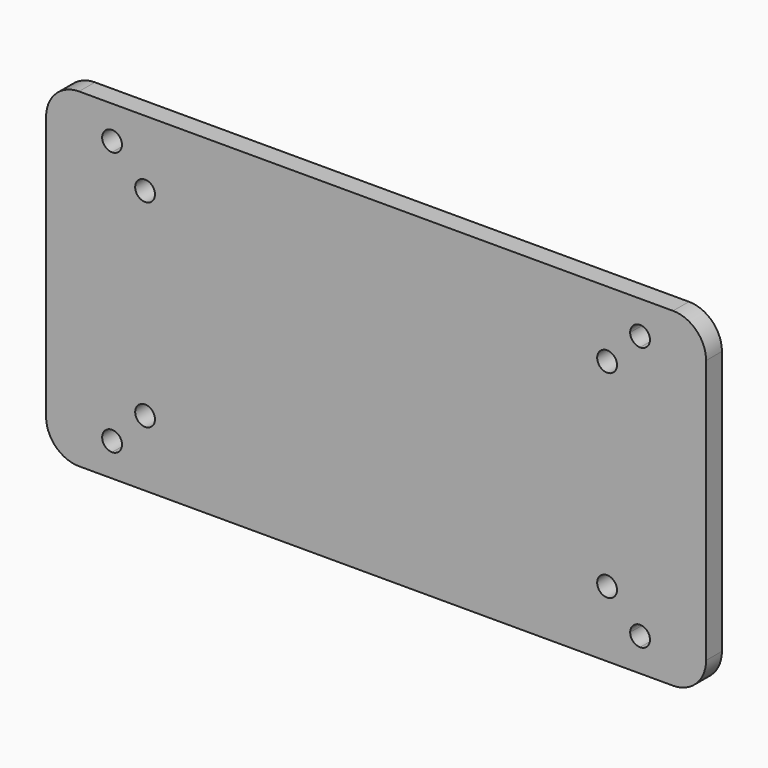
from build123d import *

# Parameters (mm, degrees)
F1_R     = 1.5
F1_R_2   = 12.8016
F2_DEPTH = 3
F3_DEPTH = 3


# Not quite as in the source:
# - a feature names something its author has since deleted; it is built from what else it names


with BuildPart() as f2:
    # F1 (on Front) → F2 (new body)
    with BuildSketch(Plane.XZ):
        with BuildLine():
            ThreePointArc((-79.8984, -48.3984), (-78.8377398282, -48.8377398282), (-78.3984, -49.8984))
            Line((-78.3984, -49.8984), (-1.3984, -49.8984))
            ThreePointArc((-1.3984, -49.8984), (-0.9590601718, -48.8377398282), (0.1016, -48.3984))
            Line((0.1016, -48.3984), (0.1016, -11.3984))
            ThreePointArc((0.1016, -11.3984), (-0.9590601718, -10.9590601718), (-1.3984, -9.8984))
            Line((-1.3984, -9.8984), (-78.3984, -9.8984))
            ThreePointArc((-78.3984, -9.8984), (-78.8377398282, -10.9590601718), (-79.8984, -11.3984))
            Line((-79.8984, -11.3984), (-79.8984, -48.3984))
        make_face()
        with Locations((-74.8984, -44.8984)):
            Circle(F1_R, mode=Mode.SUBTRACT)
        with BuildLine():
            ThreePointArc((-35.3196263313, -48.5484), (-35.6125195501, -49.2555067812), (-36.3196263313, -49.5484))
            Line((-36.3196263313, -49.5484), (-47.2771736687, -49.5484))
            ThreePointArc((-47.2771736687, -49.5484), (-47.9842804499, -49.2555067812), (-48.2771736687, -48.5484))
            Line((-48.2771736687, -48.5484), (-48.2771736687, -36.5484))
            ThreePointArc((-48.2771736687, -36.5484), (-47.9842804499, -35.8412932188), (-47.2771736687, -35.5484))
            Line((-47.2771736687, -35.5484), (-36.3196263313, -35.5484))
            ThreePointArc((-36.3196263313, -35.5484), (-35.6125195501, -35.8412932188), (-35.3196263313, -36.5484))
            Line((-35.3196263313, -36.5484), (-35.3196263313, -48.5484))
        make_face(mode=Mode.SUBTRACT)
        with Locations((-64.6584, -30.8484)):
            Circle(F1_R_2, mode=Mode.SUBTRACT)
        with Locations((-4.8984, -44.8984)):
            Circle(F1_R, mode=Mode.SUBTRACT)
        with Locations((-74.8984, -14.8984)):
            Circle(F1_R, mode=Mode.SUBTRACT)
        with BuildLine():
            ThreePointArc((-35.3196263313, -23.1484), (-35.6125195501, -23.8555067812), (-36.3196263313, -24.1484))
            Line((-36.3196263313, -24.1484), (-47.2771736687, -24.1484))
            ThreePointArc((-47.2771736687, -24.1484), (-47.9842804499, -23.8555067812), (-48.2771736687, -23.1484))
            Line((-48.2771736687, -23.1484), (-48.2771736687, -11.1484))
            ThreePointArc((-48.2771736687, -11.1484), (-47.9842804499, -10.4412932188), (-47.2771736687, -10.1484))
            Line((-47.2771736687, -10.1484), (-36.3196263313, -10.1484))
            ThreePointArc((-36.3196263313, -10.1484), (-35.6125195501, -10.4412932188), (-35.3196263313, -11.1484))
            Line((-35.3196263313, -11.1484), (-35.3196263313, -23.1484))
        make_face(mode=Mode.SUBTRACT)
        with BuildLine():
            ThreePointArc((-24.0503456444, -32.5784), (-24.3432388632, -33.2855067812), (-25.0503456444, -33.5784))
            Line((-25.0503456444, -33.5784), (-30.0664543556, -33.5784))
            ThreePointArc((-30.0664543556, -33.5784), (-30.7735611368, -33.2855067812), (-31.0664543556, -32.5784))
            Line((-31.0664543556, -32.5784), (-31.0664543556, -26.5784))
            ThreePointArc((-31.0664543556, -26.5784), (-30.7735611368, -25.8712932188), (-30.0664543556, -25.5784))
            Line((-30.0664543556, -25.5784), (-25.0503456444, -25.5784))
            ThreePointArc((-25.0503456444, -25.5784), (-24.3432388632, -25.8712932188), (-24.0503456444, -26.5784))
            Line((-24.0503456444, -26.5784), (-24.0503456444, -32.5784))
        make_face(mode=Mode.SUBTRACT)
        with BuildLine():
            ThreePointArc((-20.0169235468, -20.9634935707), (-19.724030328, -20.2563867895), (-19.0169235468, -19.9634935707))
            Line((-19.0169235468, -19.9634935707), (-13.3099917546, -19.9634935707))
            ThreePointArc((-13.3099917546, -19.9634935707), (-12.6028849734, -20.2563867895), (-12.3099917546, -20.9634935707))
            Line((-12.3099917546, -20.9634935707), (-12.3099917546, -38.3518991768))
            ThreePointArc((-12.3099917546, -38.3518991768), (-12.6028849734, -39.059005958), (-13.3099917546, -39.3518991768))
            Line((-13.3099917546, -39.3518991768), (-19.0169235468, -39.3518991768))
            ThreePointArc((-19.0169235468, -39.3518991768), (-19.724030328, -39.059005958), (-20.0169235468, -38.3518991768))
            Line((-20.0169235468, -38.3518991768), (-20.0169235468, -20.9634935707))
        make_face(mode=Mode.SUBTRACT)
        with Locations((-4.8984, -14.8984)):
            Circle(F1_R, mode=Mode.SUBTRACT)
        with BuildLine():
            Line((-79.8984, -6.8984), (-79.8984, -8.3984))
            ThreePointArc((-79.8984, -8.3984), (-78.8377398282, -8.8377398282), (-78.3984, -9.8984))
            Line((-78.3984, -9.8984), (-1.3984, -9.8984))
            ThreePointArc((-1.3984, -9.8984), (-0.9590601718, -8.8377398282), (0.1016, -8.3984))
            Line((0.1016, -8.3984), (0.1016, -6.8984))
            Line((0.1016, -6.8984), (-79.8984, -6.8984))
        make_face()
        with BuildLine():
            Line((-1.3984, -49.8984), (-78.3984, -49.8984))
            ThreePointArc((-78.3984, -49.8984), (-78.8377398282, -50.9590601718), (-79.8984, -51.3984))
            Line((-79.8984, -51.3984), (-79.8984, -52.8984))
            Line((-79.8984, -52.8984), (0.1016, -52.8984))
            Line((0.1016, -52.8984), (0.1016, -51.3984))
            ThreePointArc((0.1016, -51.3984), (-0.9590601718, -50.9590601718), (-1.3984, -49.8984))
        make_face()
    extrude(amount=F2_DEPTH)


with BuildPart() as f3:
    # F1 (on Front) → F3 (new body)
    with BuildSketch(Plane.XZ):
        with BuildLine():
            Line((-84.8984, -54.8984), (5.1016, -54.8984))
            ThreePointArc((5.1016, -54.8984), (8.6371339059, -53.4339339059), (10.1016, -49.8984))
            Line((10.1016, -49.8984), (10.1016, -9.8984))
            ThreePointArc((10.1016, -9.8984), (8.6371339059, -6.3628660941), (5.1016, -4.8984))
            Line((5.1016, -4.8984), (-84.8984, -4.8984))
            ThreePointArc((-84.8984, -4.8984), (-88.4339339059, -6.3628660941), (-89.8984, -9.8984))
            Line((-89.8984, -9.8984), (-89.8984, -49.8984))
            ThreePointArc((-89.8984, -49.8984), (-88.4339339059, -53.4339339059), (-84.8984, -54.8984))
        make_face()
        with BuildLine():
            ThreePointArc((-79.8984, -51.3984), (-81.3984, -49.8984), (-79.8984, -48.3984))
            Line((-79.8984, -48.3984), (-79.8984, -11.3984))
            ThreePointArc((-79.8984, -11.3984), (-81.3984, -9.8984), (-79.8984, -8.3984))
            Line((-79.8984, -8.3984), (-79.8984, -6.8984))
            Line((-79.8984, -6.8984), (0.1016, -6.8984))
            Line((0.1016, -6.8984), (0.1016, -8.3984))
            ThreePointArc((0.1016, -8.3984), (1.1622601718, -8.8377398282), (1.6016, -9.8984))
            ThreePointArc((1.6016, -9.8984), (1.1622601718, -10.9590601718), (0.1016, -11.3984))
            Line((0.1016, -11.3984), (0.1016, -48.3984))
            ThreePointArc((0.1016, -48.3984), (1.1622601718, -48.8377398282), (1.6016, -49.8984))
            ThreePointArc((1.6016, -49.8984), (1.1622601718, -50.9590601718), (0.1016, -51.3984))
            Line((0.1016, -51.3984), (0.1016, -52.8984))
            Line((0.1016, -52.8984), (-79.8984, -52.8984))
            Line((-79.8984, -52.8984), (-79.8984, -51.3984))
        make_face(mode=Mode.SUBTRACT)
        with BuildLine():
            ThreePointArc((-79.8984, -48.3984), (-78.8377398282, -48.8377398282), (-78.3984, -49.8984))
            Line((-78.3984, -49.8984), (-1.3984, -49.8984))
            ThreePointArc((-1.3984, -49.8984), (-0.9590601718, -48.8377398282), (0.1016, -48.3984))
            Line((0.1016, -48.3984), (0.1016, -11.3984))
            ThreePointArc((0.1016, -11.3984), (-0.9590601718, -10.9590601718), (-1.3984, -9.8984))
            Line((-1.3984, -9.8984), (-78.3984, -9.8984))
            ThreePointArc((-78.3984, -9.8984), (-78.8377398282, -10.9590601718), (-79.8984, -11.3984))
            Line((-79.8984, -11.3984), (-79.8984, -48.3984))
        make_face()
        with Locations((-74.8984, -44.8984)):
            Circle(F1_R, mode=Mode.SUBTRACT)
        with BuildLine():
            ThreePointArc((-35.3196263313, -48.5484), (-35.6125195501, -49.2555067812), (-36.3196263313, -49.5484))
            Line((-36.3196263313, -49.5484), (-47.2771736687, -49.5484))
            ThreePointArc((-47.2771736687, -49.5484), (-47.9842804499, -49.2555067812), (-48.2771736687, -48.5484))
            Line((-48.2771736687, -48.5484), (-48.2771736687, -36.5484))
            ThreePointArc((-48.2771736687, -36.5484), (-47.9842804499, -35.8412932188), (-47.2771736687, -35.5484))
            Line((-47.2771736687, -35.5484), (-36.3196263313, -35.5484))
            ThreePointArc((-36.3196263313, -35.5484), (-35.6125195501, -35.8412932188), (-35.3196263313, -36.5484))
            Line((-35.3196263313, -36.5484), (-35.3196263313, -48.5484))
        make_face(mode=Mode.SUBTRACT)
        with Locations((-64.6584, -30.8484)):
            Circle(F1_R_2, mode=Mode.SUBTRACT)
        with Locations((-4.8984, -44.8984)):
            Circle(F1_R, mode=Mode.SUBTRACT)
        with Locations((-74.8984, -14.8984)):
            Circle(F1_R, mode=Mode.SUBTRACT)
        with BuildLine():
            ThreePointArc((-35.3196263313, -23.1484), (-35.6125195501, -23.8555067812), (-36.3196263313, -24.1484))
            Line((-36.3196263313, -24.1484), (-47.2771736687, -24.1484))
            ThreePointArc((-47.2771736687, -24.1484), (-47.9842804499, -23.8555067812), (-48.2771736687, -23.1484))
            Line((-48.2771736687, -23.1484), (-48.2771736687, -11.1484))
            ThreePointArc((-48.2771736687, -11.1484), (-47.9842804499, -10.4412932188), (-47.2771736687, -10.1484))
            Line((-47.2771736687, -10.1484), (-36.3196263313, -10.1484))
            ThreePointArc((-36.3196263313, -10.1484), (-35.6125195501, -10.4412932188), (-35.3196263313, -11.1484))
            Line((-35.3196263313, -11.1484), (-35.3196263313, -23.1484))
        make_face(mode=Mode.SUBTRACT)
        with BuildLine():
            ThreePointArc((-24.0503456444, -32.5784), (-24.3432388632, -33.2855067812), (-25.0503456444, -33.5784))
            Line((-25.0503456444, -33.5784), (-30.0664543556, -33.5784))
            ThreePointArc((-30.0664543556, -33.5784), (-30.7735611368, -33.2855067812), (-31.0664543556, -32.5784))
            Line((-31.0664543556, -32.5784), (-31.0664543556, -26.5784))
            ThreePointArc((-31.0664543556, -26.5784), (-30.7735611368, -25.8712932188), (-30.0664543556, -25.5784))
            Line((-30.0664543556, -25.5784), (-25.0503456444, -25.5784))
            ThreePointArc((-25.0503456444, -25.5784), (-24.3432388632, -25.8712932188), (-24.0503456444, -26.5784))
            Line((-24.0503456444, -26.5784), (-24.0503456444, -32.5784))
        make_face(mode=Mode.SUBTRACT)
        with BuildLine():
            ThreePointArc((-20.0169235468, -20.9634935707), (-19.724030328, -20.2563867895), (-19.0169235468, -19.9634935707))
            Line((-19.0169235468, -19.9634935707), (-13.3099917546, -19.9634935707))
            ThreePointArc((-13.3099917546, -19.9634935707), (-12.6028849734, -20.2563867895), (-12.3099917546, -20.9634935707))
            Line((-12.3099917546, -20.9634935707), (-12.3099917546, -38.3518991768))
            ThreePointArc((-12.3099917546, -38.3518991768), (-12.6028849734, -39.059005958), (-13.3099917546, -39.3518991768))
            Line((-13.3099917546, -39.3518991768), (-19.0169235468, -39.3518991768))
            ThreePointArc((-19.0169235468, -39.3518991768), (-19.724030328, -39.059005958), (-20.0169235468, -38.3518991768))
            Line((-20.0169235468, -38.3518991768), (-20.0169235468, -20.9634935707))
        make_face(mode=Mode.SUBTRACT)
        with Locations((-4.8984, -14.8984)):
            Circle(F1_R, mode=Mode.SUBTRACT)
        with Locations((-64.6584, -30.8484)):
            Circle(F1_R_2)
        with BuildLine():
            Line((-79.8984, -6.8984), (-79.8984, -8.3984))
            ThreePointArc((-79.8984, -8.3984), (-78.8377398282, -8.8377398282), (-78.3984, -9.8984))
            Line((-78.3984, -9.8984), (-1.3984, -9.8984))
            ThreePointArc((-1.3984, -9.8984), (-0.9590601718, -8.8377398282), (0.1016, -8.3984))
            Line((0.1016, -8.3984), (0.1016, -6.8984))
            Line((0.1016, -6.8984), (-79.8984, -6.8984))
        make_face()
        with BuildLine():
            Line((-1.3984, -49.8984), (-78.3984, -49.8984))
            ThreePointArc((-78.3984, -49.8984), (-78.8377398282, -50.9590601718), (-79.8984, -51.3984))
            Line((-79.8984, -51.3984), (-79.8984, -52.8984))
            Line((-79.8984, -52.8984), (0.1016, -52.8984))
            Line((0.1016, -52.8984), (0.1016, -51.3984))
            ThreePointArc((0.1016, -51.3984), (-0.9590601718, -50.9590601718), (-1.3984, -49.8984))
        make_face()
        with BuildLine():
            Line((-47.2771736687, -24.1484), (-36.3196263313, -24.1484))
            ThreePointArc((-36.3196263313, -24.1484), (-35.6125195501, -23.8555067812), (-35.3196263313, -23.1484))
            Line((-35.3196263313, -23.1484), (-35.3196263313, -11.1484))
            ThreePointArc((-35.3196263313, -11.1484), (-35.6125195501, -10.4412932188), (-36.3196263313, -10.1484))
            Line((-36.3196263313, -10.1484), (-47.2771736687, -10.1484))
            ThreePointArc((-47.2771736687, -10.1484), (-47.9842804499, -10.4412932188), (-48.2771736687, -11.1484))
            Line((-48.2771736687, -11.1484), (-48.2771736687, -23.1484))
            ThreePointArc((-48.2771736687, -23.1484), (-47.9842804499, -23.8555067812), (-47.2771736687, -24.1484))
        make_face()
        with BuildLine():
            Line((-47.2771736687, -49.5484), (-36.3196263313, -49.5484))
            ThreePointArc((-36.3196263313, -49.5484), (-35.6125195501, -49.2555067812), (-35.3196263313, -48.5484))
            Line((-35.3196263313, -48.5484), (-35.3196263313, -36.5484))
            ThreePointArc((-35.3196263313, -36.5484), (-35.6125195501, -35.8412932188), (-36.3196263313, -35.5484))
            Line((-36.3196263313, -35.5484), (-47.2771736687, -35.5484))
            ThreePointArc((-47.2771736687, -35.5484), (-47.9842804499, -35.8412932188), (-48.2771736687, -36.5484))
            Line((-48.2771736687, -36.5484), (-48.2771736687, -48.5484))
            ThreePointArc((-48.2771736687, -48.5484), (-47.9842804499, -49.2555067812), (-47.2771736687, -49.5484))
        make_face()
        with BuildLine():
            Line((-13.3099917546, -19.9634935707), (-19.0169235468, -19.9634935707))
            ThreePointArc((-19.0169235468, -19.9634935707), (-19.724030328, -20.2563867895), (-20.0169235468, -20.9634935707))
            Line((-20.0169235468, -20.9634935707), (-20.0169235468, -38.3518991768))
            ThreePointArc((-20.0169235468, -38.3518991768), (-19.724030328, -39.059005958), (-19.0169235468, -39.3518991768))
            Line((-19.0169235468, -39.3518991768), (-13.3099917546, -39.3518991768))
            ThreePointArc((-13.3099917546, -39.3518991768), (-12.6028849734, -39.059005958), (-12.3099917546, -38.3518991768))
            Line((-12.3099917546, -38.3518991768), (-12.3099917546, -20.9634935707))
            ThreePointArc((-12.3099917546, -20.9634935707), (-12.6028849734, -20.2563867895), (-13.3099917546, -19.9634935707))
        make_face()
        with BuildLine():
            Line((-30.0664543556, -33.5784), (-25.0503456444, -33.5784))
            ThreePointArc((-25.0503456444, -33.5784), (-24.3432388632, -33.2855067812), (-24.0503456444, -32.5784))
            Line((-24.0503456444, -32.5784), (-24.0503456444, -26.5784))
            ThreePointArc((-24.0503456444, -26.5784), (-24.3432388632, -25.8712932188), (-25.0503456444, -25.5784))
            Line((-25.0503456444, -25.5784), (-30.0664543556, -25.5784))
            ThreePointArc((-30.0664543556, -25.5784), (-30.7735611368, -25.8712932188), (-31.0664543556, -26.5784))
            Line((-31.0664543556, -26.5784), (-31.0664543556, -32.5784))
            ThreePointArc((-31.0664543556, -32.5784), (-30.7735611368, -33.2855067812), (-30.0664543556, -33.5784))
        make_face()
    extrude(amount=F3_DEPTH)


solid = Compound([f2.part, f3.part])
